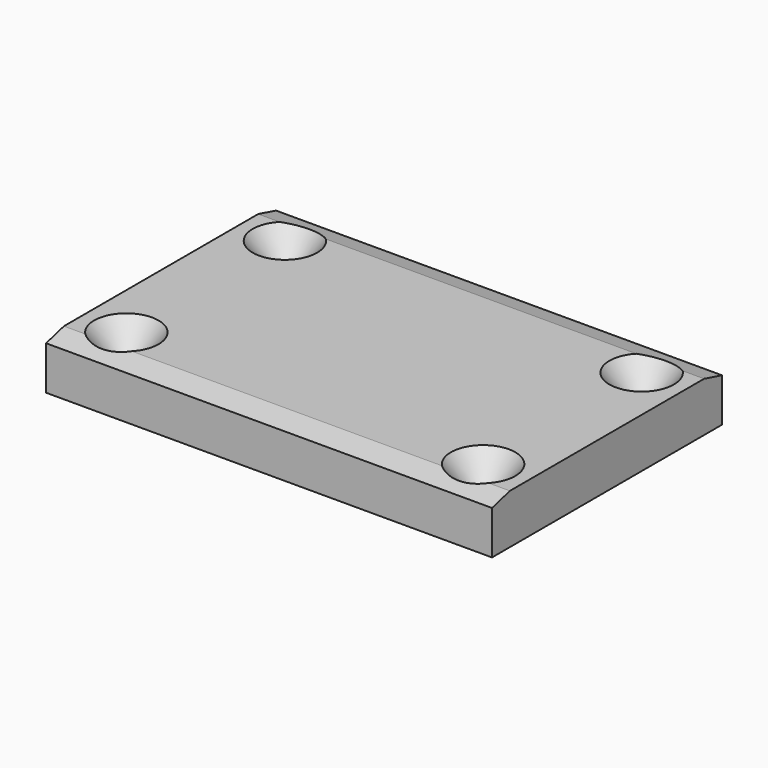
from build123d import *

# Parameters (mm, degrees)
F0_W        = 180
F0_H        = 116
F0_R        = 5.25
F1_DEPTH    = 20
F2_SIZE2    = 7.75
F2_SIZE     = 10
F2_2_SIZE2  = 7.75
F2_2_SIZE   = 10
F2_3_SIZE2  = 7.75
F2_3_SIZE   = 10
F2_4_SIZE2  = 7.75
F2_4_SIZE   = 10
F3_T1_DEPTH = 226.7409882636


# Not quite as in the source:
# - a fillet or chamfer that OpenCascade refuses, or shapes differently, is made with other operations: its cross-section is extruded or revolved along the edge and cut away or added


with BuildPart() as f1:
    # F0 (on Top) → F1 (new body)
    with BuildSketch(Plane.XY):
        with Locations((-6.8610161543, -3.4973233796)):
            Rectangle(F0_W, F0_H)
        with Locations((-78.8610161543, -43.4973233796)):
            Circle(F0_R, mode=Mode.SUBTRACT)
        with Locations((65.1389838457, -43.4973233796)):
            Circle(F0_R, mode=Mode.SUBTRACT)
        with Locations((-78.8610161543, 36.5026766204)):
            Circle(F0_R, mode=Mode.SUBTRACT)
        with Locations((65.1389838457, 36.5026766204)):
            Circle(F0_R, mode=Mode.SUBTRACT)
    extrude(amount=F1_DEPTH)

    # F2
    f2_edges = [f1.edges().sort_by_distance(p)[0] for p in [
        (59.888984, -43.497323, 20),
    ]]
    f2_side = f1.faces().sort_by_distance((59.888984, -43.497323, 10))[0]
    chamfer(f2_edges, length=F2_SIZE, length2=F2_SIZE2, reference=f2_side)

    # F2#2
    f2_2_edges = [f1.edges().sort_by_distance(p)[0] for p in [
        (-84.111016, -43.497323, 20),
    ]]
    f2_2_side = f1.faces().sort_by_distance((-84.111016, -43.497323, 10))[0]
    chamfer(f2_2_edges, length=F2_2_SIZE, length2=F2_2_SIZE2, reference=f2_2_side)

    # F2#3
    f2_3_edges = [f1.edges().sort_by_distance(p)[0] for p in [
        (-84.111016, 36.502677, 20),
    ]]
    f2_3_side = f1.faces().sort_by_distance((-84.111016, 36.502677, 10))[0]
    chamfer(f2_3_edges, length=F2_3_SIZE, length2=F2_3_SIZE2, reference=f2_3_side)

    # F2#4
    f2_4_edges = [f1.edges().sort_by_distance(p)[0] for p in [
        (59.888984, 36.502677, 20),
    ]]
    f2_4_side = f1.faces().sort_by_distance((59.888984, 36.502677, 10))[0]
    chamfer(f2_4_edges, length=F2_4_SIZE, length2=F2_4_SIZE2, reference=f2_4_side)

    # F3: chamfer of 9 x 2.4115427319 on 2 edges, made by hand

    # F3_s2 → F3_t1 (cut)
    with BuildSketch(Plane.YZ.offset(-120.2315102861)):
        Polygon((-52.4973233796, 20), (-61.4973233796, 17.5884572681), (-61.4973233796, 20), align=None)
        Polygon((45.5026766204, 20), (54.5026766204, 17.5884572681), (54.5026766204, 20), align=None)
    extrude(amount=F3_T1_DEPTH, mode=Mode.SUBTRACT)


solid = f1.part
